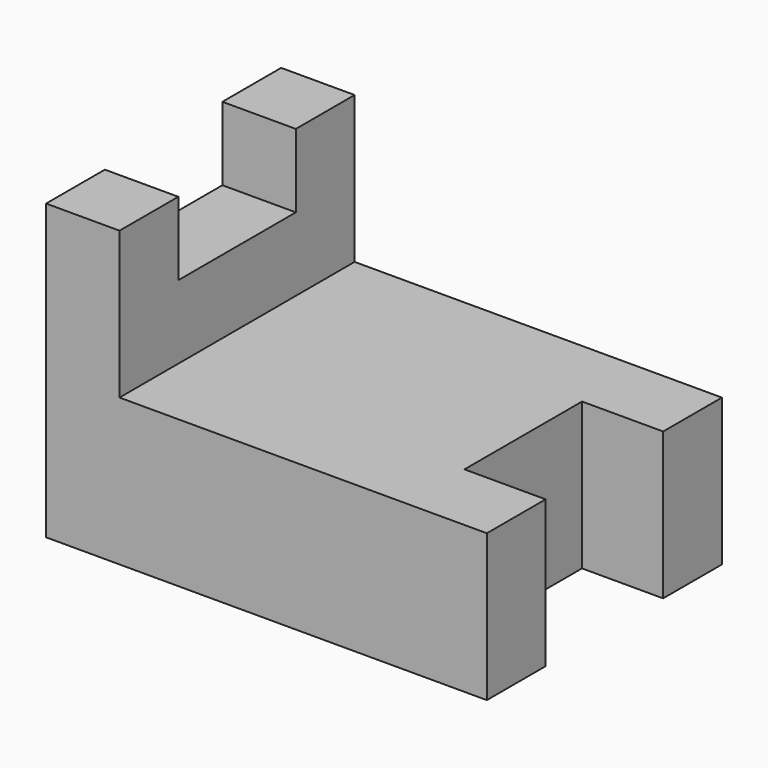
from build123d import *

# Parameters (mm, degrees)
F1_DEPTH = 25.4
F2_W     = 6.35
F2_H     = 12.7
F3_DEPTH = 6.35
F4_W     = 7.0131157884
F4_H     = 12.7
F5_DEPTH = 12.7


# Not quite as in the source:
# - a feature names something its author has since deleted; it is built from what else it names


with BuildPart() as f1:
    # F0 (on Front) → F1 (new body)
    with BuildSketch(Plane.XZ):
        Polygon((6.35, 25.4), (0, 25.4), (0, 0), (38.1, 0), (38.1, 12.7), (6.35, 12.7), align=None)
    extrude(amount=F1_DEPTH)

    # F2 (on face) → F3 (cut)
    with BuildSketch(Plane.XY.offset(25.4)):
        with Locations((3.175, -12.7)):
            Rectangle(F2_W, F2_H)
    extrude(amount=-F3_DEPTH, mode=Mode.SUBTRACT)

    # F4 (on face) → F5 (cut)
    with BuildSketch(Plane.XY.offset(12.7)):
        with Locations((34.5934421058, -12.7)):
            Rectangle(F4_W, F4_H)
    extrude(amount=-F5_DEPTH, mode=Mode.SUBTRACT)


solid = f1.part
